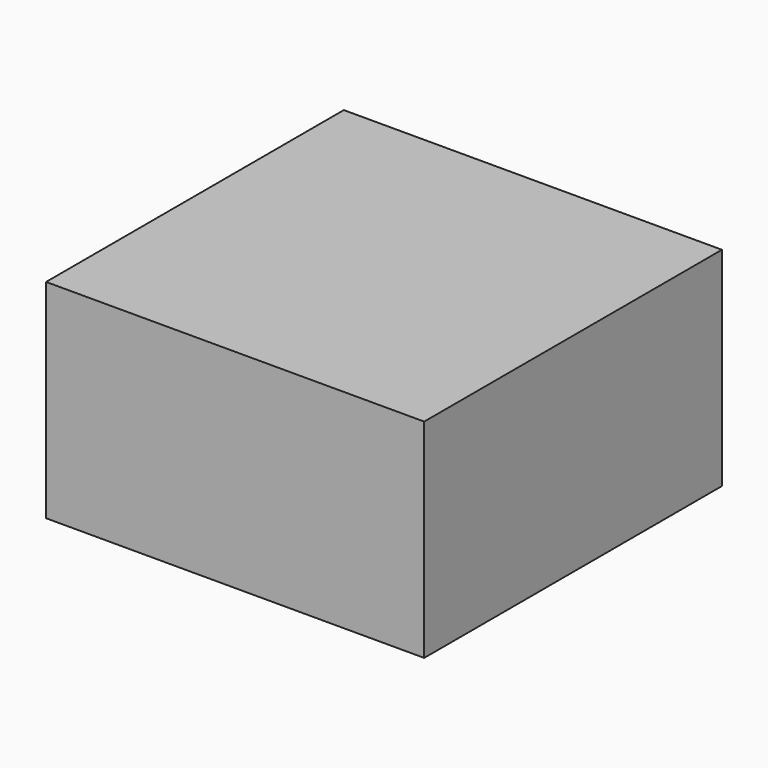
from build123d import *

# Parameters (mm, degrees)
F0_W     = 69.8630958796
F0_H     = 137.5265717506
F2_DEPTH = 76.8858


# Not quite as in the source:
# - the program builds the solid bodies; features that only make, move or delete a surface that nothing else refers to are left out


with BuildPart() as f2:
    # F0 (on Top) → F2 (new body)
    with BuildSketch(Plane.XY):
        with Locations((-34.9315479398, 0)):
            Rectangle(F0_W, F0_H)
        with Locations((34.9315479398, 0)):
            Rectangle(F0_W, F0_H)
    extrude(amount=-F2_DEPTH)


solid = f2.part
